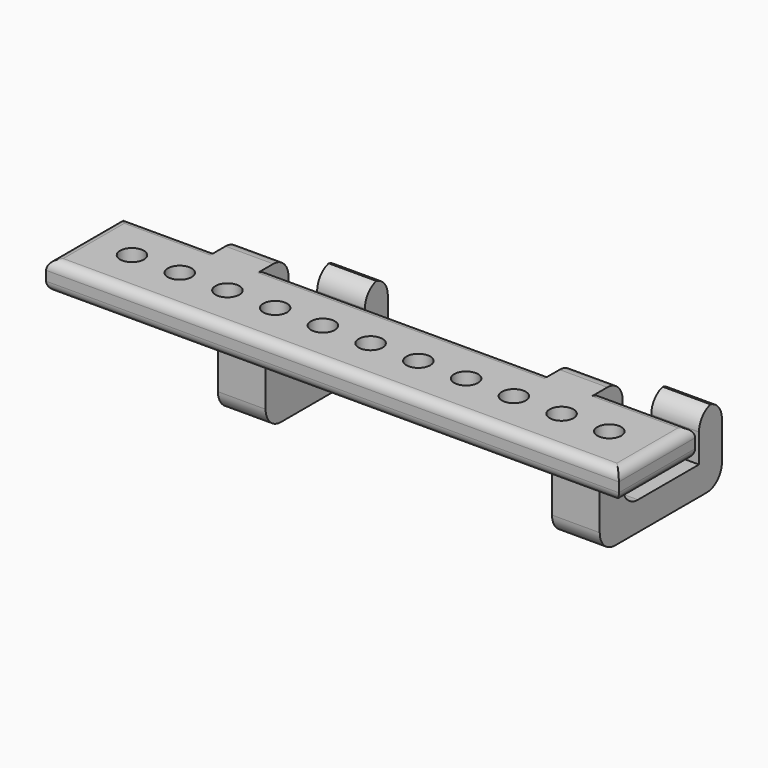
from build123d import *

# Parameters (mm, degrees)
F0_W        = 60
F0_H        = 10
F1_DEPTH    = 3
F2_R        = 1.25
F3_DEPTH    = 3
F4_W        = 5
F4_H        = 15
F5_DEPTH    = 16
F7_DEPTH    = 60
F8_T1_DEPTH = 5
F8_T3_DEPTH = 5
F8_T5_DEPTH = 15
F8_T7_DEPTH = 15
F9_R        = 1


# Not quite as in the source:
# - a fillet or chamfer that OpenCascade refuses, or shapes differently, is made with other operations: its cross-section is extruded or revolved along the edge and cut away or added


with BuildPart() as f1:
    # F0 (on Top) → F1 (new body)
    with BuildSketch(Plane.XY):
        Rectangle(F0_W, F0_H)
    extrude(amount=F1_DEPTH)

    # F2 (on face) → F3 (cut)
    with BuildSketch(Plane.XY.offset(3)):
        with Locations((-25, 0)):
            Circle(F2_R)
        with Locations((-20, 0)):
            Circle(F2_R)
        with Locations((-15, 0)):
            Circle(F2_R)
        with Locations((-10, 0)):
            Circle(F2_R)
        with Locations((-5, 0)):
            Circle(F2_R)
        Circle(F2_R)
        with Locations((5, 0)):
            Circle(F2_R)
        with Locations((10, 0)):
            Circle(F2_R)
        with Locations((15, 0)):
            Circle(F2_R)
        with Locations((20, 0)):
            Circle(F2_R)
        with Locations((25, 0)):
            Circle(F2_R)
    extrude(amount=-F3_DEPTH, mode=Mode.SUBTRACT)

    # F4 (on face) → F5 (join)
    with BuildSketch(Plane(origin=(0, 5, 0), x_dir=(-1, 0, 0), z_dir=(0, 1, 0))):
        with Locations((17.5, -4.5)):
            Rectangle(F4_W, F4_H)
        with Locations((-17.5, -4.5)):
            Rectangle(F4_W, F4_H)
    extrude(amount=F5_DEPTH)

    # F6 (on face) → F7 (cut)
    with BuildSketch(Plane(origin=(-20, 0, 0), x_dir=(0, -1, 0), z_dir=(-1, 0, 0))):
        Polygon((-8, -9), (-8, 3), (-21, 3), (-21, -4), (-18, -4), (-18, -9), align=None)
    extrude(amount=-F7_DEPTH, mode=Mode.SUBTRACT)

    # F8: fillet of radius 2 on 17 edges, made by hand

    # F8_s2 → F8_t1 (join)
    with BuildSketch(Plane.YZ.offset(15)):
        with BuildLine():
            ThreePointArc((3, 0), (4.4142135624, -0.5857864376), (5, -2))
            Line((5, -2), (5, 0))
            Line((5, 0), (3, 0))
        make_face()
        with BuildLine():
            ThreePointArc((10, -9), (8.5857864376, -8.4142135624), (8, -7))
            Line((8, -7), (8, -9))
            Line((8, -9), (10, -9))
        make_face()
    extrude(amount=F8_T1_DEPTH)

    # F8_s4 → F8_t3 (join)
    with BuildSketch(Plane.YZ.offset(-20)):
        with BuildLine():
            ThreePointArc((3, 0), (4.4142135624, -0.5857864376), (5, -2))
            Line((5, -2), (5, 0))
            Line((5, 0), (3, 0))
        make_face()
        with BuildLine():
            ThreePointArc((8, -7), (8.5857864376, -8.4142135624), (10, -9))
            Line((10, -9), (8, -9))
            Line((8, -9), (8, -7))
        make_face()
    extrude(amount=F8_T3_DEPTH)

    # F8_s6 → F8_t5 (cut)
    with BuildSketch(Plane.YZ.offset(-25)):
        with BuildLine():
            ThreePointArc((5, -10), (5.5857864376, -11.4142135624), (7, -12))
            Line((7, -12), (5, -12))
            Line((5, -12), (5, -10))
        make_face()
        with BuildLine():
            ThreePointArc((21, -10), (20.4142135624, -11.4142135624), (19, -12))
            Line((19, -12), (21, -12))
            Line((21, -12), (21, -10))
        make_face()
        with BuildLine():
            ThreePointArc((19, -4), (20.4142135624, -4.5857864376), (21, -6))
            Line((21, -6), (21, -4))
            Line((21, -4), (19, -4))
        make_face()
        with BuildLine():
            ThreePointArc((18, -6), (18.5857864376, -4.5857864376), (20, -4))
            Line((20, -4), (18, -4))
            Line((18, -4), (18, -6))
        make_face()
        with BuildLine():
            ThreePointArc((6, 3), (7.4142135624, 2.4142135624), (8, 1))
            Line((8, 1), (8, 3))
            Line((8, 3), (6, 3))
        make_face()
    extrude(amount=F8_T5_DEPTH, mode=Mode.SUBTRACT)

    # F8_s8 → F8_t7 (cut)
    with BuildSketch(Plane.YZ.offset(10)):
        with BuildLine():
            ThreePointArc((5, -10), (5.5857864376, -11.4142135624), (7, -12))
            Line((7, -12), (5, -12))
            Line((5, -12), (5, -10))
        make_face()
        with BuildLine():
            ThreePointArc((19, -12), (20.4142135624, -11.4142135624), (21, -10))
            Line((21, -10), (21, -12))
            Line((21, -12), (19, -12))
        make_face()
        with BuildLine():
            ThreePointArc((21, -6), (20.4142135624, -4.5857864376), (19, -4))
            Line((19, -4), (21, -4))
            Line((21, -4), (21, -6))
        make_face()
        with BuildLine():
            ThreePointArc((20, -4), (18.5857864376, -4.5857864376), (18, -6))
            Line((18, -6), (18, -4))
            Line((18, -4), (20, -4))
        make_face()
        with BuildLine():
            ThreePointArc((6, 3), (7.4142135624, 2.4142135624), (8, 1))
            Line((8, 1), (8, 3))
            Line((8, 3), (6, 3))
        make_face()
    extrude(amount=F8_T7_DEPTH, mode=Mode.SUBTRACT)

    # F9
    f9_edges = [f1.edges().sort_by_distance(p)[0] for p in [
        (0, -5, 3),
        (30, 0, 3),
        (25, 5, 3),
        (0, 5, 3),
        (-25, 5, 3),
        (-30, 0, 3),
        (0, -5, 0),
        (30, 0, 0),
        (25, 5, 0),
        (0, 5, 0),
        (-25, 5, 0),
        (-30, 0, 0),
    ]]
    fillet(f9_edges, radius=F9_R)


solid = f1.part
